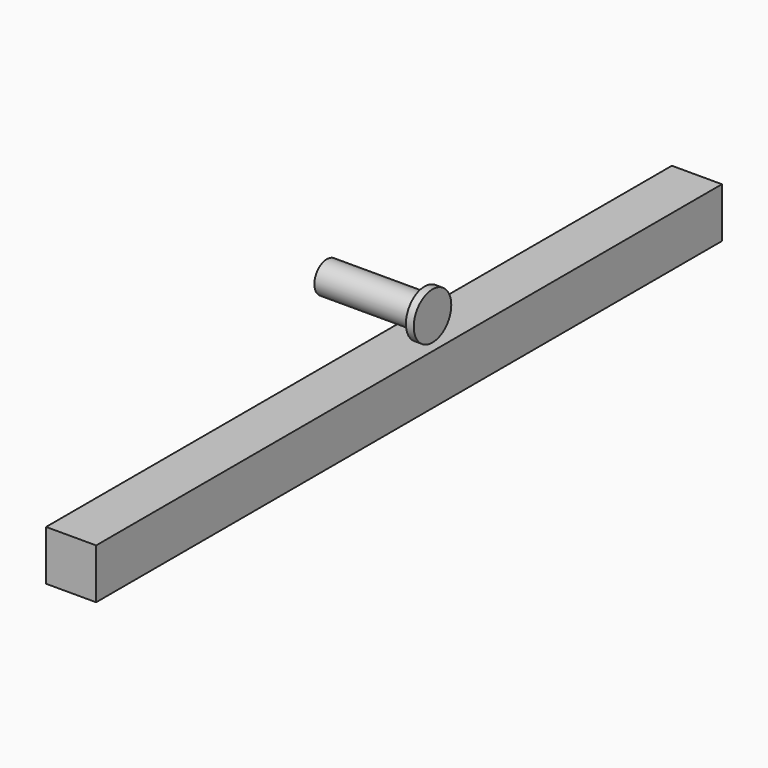
from build123d import *

# Parameters (mm, degrees)
F0_R      = 6
F1_DEPTH  = 2
F2_R      = 4
F3_DEPTH  = 25
F9_W      = 12.8
F9_H      = 12.8
F10_DEPTH = 100
F11_DEPTH = 200


# Not quite as in the source:
# - the program builds the solid bodies; features that only make, move or delete a surface that nothing else refers to are left out


with BuildPart() as f1:
    # F0 (on Right) → F1 (new body)
    with BuildSketch(Plane.YZ):
        Circle(F0_R)
    extrude(amount=F1_DEPTH)

    # F2 (on Right) → F3 (join)
    with BuildSketch(Plane.YZ):
        Circle(F2_R)
    extrude(amount=-F3_DEPTH)


with BuildPart() as f10:
    # F9 (on Front) → F10 (new body)
    with BuildSketch(Plane.XZ):
        with Locations((-10.4, -19.3641381563)):
            Rectangle(F9_W, F9_H)
    extrude(amount=F10_DEPTH)

    # F11 (add): a face of the model
    f11_faces = [f10.faces().sort_by_distance(p)[0] for p in [
        (-10.4, -100, -19.3641381563),
    ]]
    extrude(f11_faces, amount=-F11_DEPTH)


solid = Compound([f1.part, f10.part])
